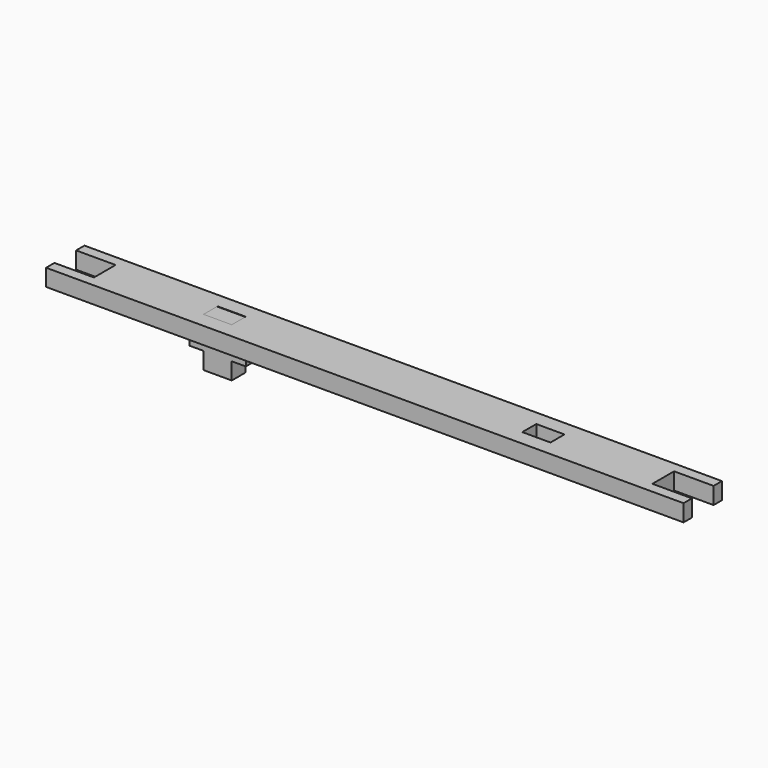
from build123d import *

# Parameters (mm, degrees)
F0_W     = 5
F0_H     = 3.1
F1_DEPTH = 3
F3_W     = 5
F3_H     = 3
F4_DEPTH = 3


# Not quite as in the source:
# - a feature names something its author has since deleted; it is built from what else it names


with BuildPart() as f1:
    # F0 (on Top) → F1 (new body)
    with BuildSketch(Plane.XY):
        Polygon((0, -4.25), (0, 4.25), (-56.5, 4.25), (-56.5, 2.4), (-49.5, 2.4), (-49.5, -2.4), (-56.5, -2.4), (-56.5, -4.25), align=None)
        with Locations((-28.25, 0)):
            Rectangle(F0_W, F0_H, mode=Mode.SUBTRACT)
    extrude(amount=F1_DEPTH)

    # F2: F1 across face


with BuildPart() as f1_1:
    add(f1.part)
    add(f1.part.mirror(Plane(origin=(0, 0, 1.5), x_dir=(0, 1, 0), z_dir=(1, 0, 0))))


with BuildPart() as f4:
    # F3 (on face) → F4 (new body)
    with BuildSketch(Plane(origin=(0, -1.55, 0), x_dir=(-1, 0, 0), z_dir=(0, 1, 0))):
        with Locations((28.25, -4.2)):
            Rectangle(F3_W, F3_H)
        Polygon((30.75, 0), (25.75, 0), (23.25, 0), (23.25, -2.7), (25.75, -2.7), (30.75, -2.7), (33.25, -2.7), (33.25, 0), align=None)
        with Locations((28.25, 1.5)):
            Rectangle(F3_W, F3_H)
    extrude(amount=F4_DEPTH)


solid = Compound([f1_1.part, f4.part])
